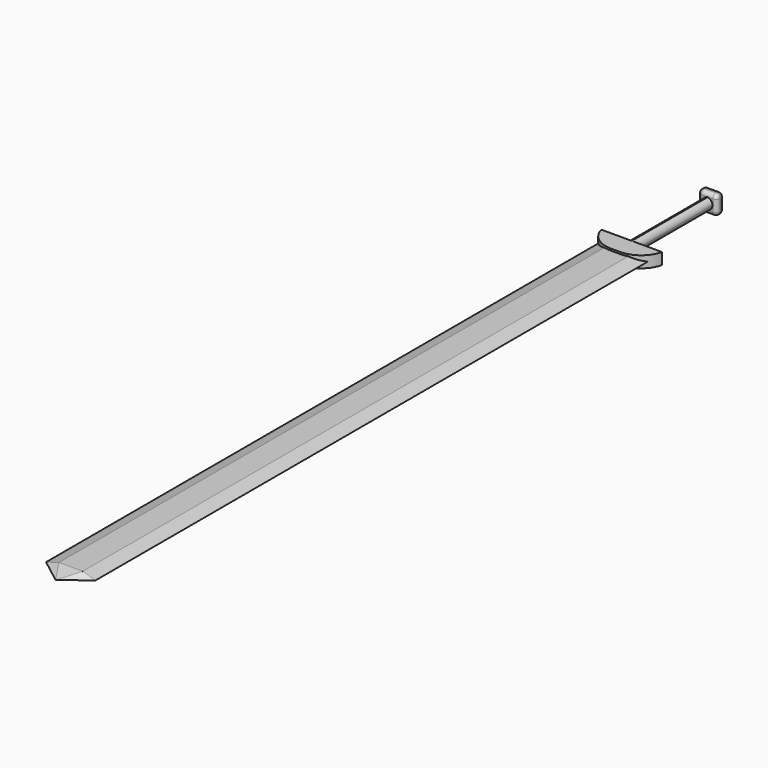
from build123d import *

# Parameters (mm, degrees)
F0_W          = 152.4
F0_H          = 15.24
F1_DEPTH      = 12.7
F2_T1_DEPTH   = 190.5
F4_W          = 25.0697992742
F4_H          = 11.7348134518
F5_DEPTH      = 12.7
F5_DEPTH_BACK = 12.7
F7_DEPTH      = 7.62
F7_DEPTH_BACK = 7.62
F8_W          = 65.6082034111
F8_H          = 914.4
F9_DEPTH      = 5.08
F9_DEPTH_BACK = 5.08
F11_DEPTH     = 914.4
F12_DEPTH     = 12.7
F16_R         = 5.08


# Not quite as in the source:
# - a fillet or chamfer that OpenCascade refuses, or shapes differently, is made with other operations: its cross-section is extruded or revolved along the edge and cut away or added


with BuildPart() as f1:
    # F0 (on Right) → F1 (new body)
    with BuildSketch(Plane.YZ):
        with Locations((76.2, -7.62)):
            Rectangle(F0_W, F0_H)
    extrude(amount=F1_DEPTH)

    # F2: fillet of radius 7.62 on 4 edges, made by hand

    # F2_s2 → F2_t1 (cut)
    with BuildSketch(Plane.XZ.offset(-171.45)):
        with BuildLine():
            ThreePointArc((7.62, 0), (2.2318463274, -2.2318463274), (0, -7.62))
            Line((0, -7.62), (0, 0))
            Line((0, 0), (7.62, 0))
        make_face()
        with BuildLine():
            ThreePointArc((7.62, -15.24), (2.2318463274, -13.0081536726), (0, -7.62))
            Line((0, -7.62), (0, -15.24))
            Line((0, -15.24), (7.62, -15.24))
        make_face()
        with BuildLine():
            ThreePointArc((5.08, 0), (10.4681536726, -2.2318463274), (12.7, -7.62))
            Line((12.7, -7.62), (12.7, 0))
            Line((12.7, 0), (5.08, 0))
        make_face()
        with BuildLine():
            ThreePointArc((5.08, -15.24), (10.4681536726, -13.0081536726), (12.7, -7.62))
            Line((12.7, -7.62), (12.7, -15.24))
            Line((12.7, -15.24), (5.08, -15.24))
        make_face()
    extrude(amount=F2_T1_DEPTH, mode=Mode.SUBTRACT)

    # F4 (on offset) → F5 (join, two sides)
    with BuildSketch(Plane.XY.offset(-7.62)) as f5_sk:
        with Locations((6.0101542622, 157.924503088)):
            Rectangle(F4_W, F4_H)
    extrude(amount=F5_DEPTH)
    extrude(f5_sk.sketch, amount=-F5_DEPTH_BACK)

    # F6 (on offset) → F7 (join, two sides)
    with BuildSketch(Plane.XY.offset(-7.62)) as f7_sk:
        with BuildLine():
            Line((6.3893780661, -0.6641601572), (12.5797659928, -0.6641601572))
            ThreePointArc((12.5797659928, -0.6641601572), (34.2227463889, 6.8879561013), (46.4923181534, 26.2505661817))
            Line((46.4923181534, 26.2505661817), (6.3893780661, 26.2505661817))
            Line((6.3893780661, 26.2505661817), (6.3893780661, -0.6641601572))
        make_face()
        with BuildLine():
            Line((0.1989901393, -0.6641601572), (6.3893780661, -0.6641601572))
            Line((6.3893780661, -0.6641601572), (6.3893780661, 26.2505661817))
            Line((6.3893780661, 26.2505661817), (-33.7397263339, 26.2505661817))
            ThreePointArc((-33.7397263339, 26.2505661817), (-21.4587969692, 6.8812254508), (0.1989901393, -0.6641601572))
        make_face()
    extrude(amount=F7_DEPTH)
    extrude(f7_sk.sketch, amount=-F7_DEPTH_BACK)

    # F8 (on offset) → F9 (join, two sides)
    with BuildSketch(Plane.XY.offset(-7.62)) as f9_sk:
        with Locations((6.5435543656, -446.0204662129)):
            Rectangle(F8_W, F8_H)
    extrude(amount=-F9_DEPTH)
    extrude(f9_sk.sketch, amount=F9_DEPTH_BACK)

    # F10 (on face) → F11 (cut)
    with BuildSketch(Plane.XZ.offset(903.2204662129)):
        Polygon((-26.2605473399, -2.54), (-26.2605473399, -7.62), (-9.2217093514, -2.54), align=None)
        Polygon((-9.2217093514, -12.7), (-26.2605473399, -7.62), (-26.2605473399, -12.7), align=None)
        Polygon((39.3476560712, -7.62), (22.3088180826, -12.7), (39.3476560712, -12.7), align=None)
        Polygon((39.3476560712, -2.54), (22.3088180826, -2.54), (39.3476560712, -7.62), align=None)
    extrude(amount=-F11_DEPTH, mode=Mode.SUBTRACT)

    # F12 (add): a face of the model
    f12_faces = [f1.faces().sort_by_distance(p)[0] for p in [
        (6.3771735992, 14.5847815456, 0),
    ]]
    extrude(f12_faces, amount=-F12_DEPTH)

    # F9_face (on face) → F15 section 0
    with BuildSketch(Plane(origin=(6.5435543656, -903.2204662129, -7.62), x_dir=(1, 0, 0), z_dir=(0, -1, 0)), mode=Mode.PRIVATE) as f15_s0:
        Polygon((-32.8041017056, 0), (-15.765263717, -5.08), (15.765263717, -5.08), (32.8041017056, 0), (15.765263717, 5.08), (-15.765263717, 5.08), align=None)
    loft([f15_s0.sketch, Vertex(6.6463528201, -928.6204662129, -7.5741349719)])

    # F16
    f16_edges = [f1.edges().sort_by_distance(p)[0] for p in [
        (-6.524745, 163.79191, -7.62),
        (-6.524745, 157.924503, 5.08),
        (-6.524745, 152.057096, -7.62),
        (-6.524745, 157.924503, -20.32),
        (6.010154, 152.057096, 5.08),
        (18.545054, 157.924503, 5.08),
        (6.010154, 163.79191, 5.08),
        (18.545054, 163.79191, -7.62),
        (18.545054, 157.924503, -20.32),
        (18.545054, 152.057096, -7.62),
        (6.010154, 152.057096, -20.32),
        (6.010154, 163.79191, -20.32),
    ]]
    fillet(f16_edges, radius=F16_R)


solid = f1.part
